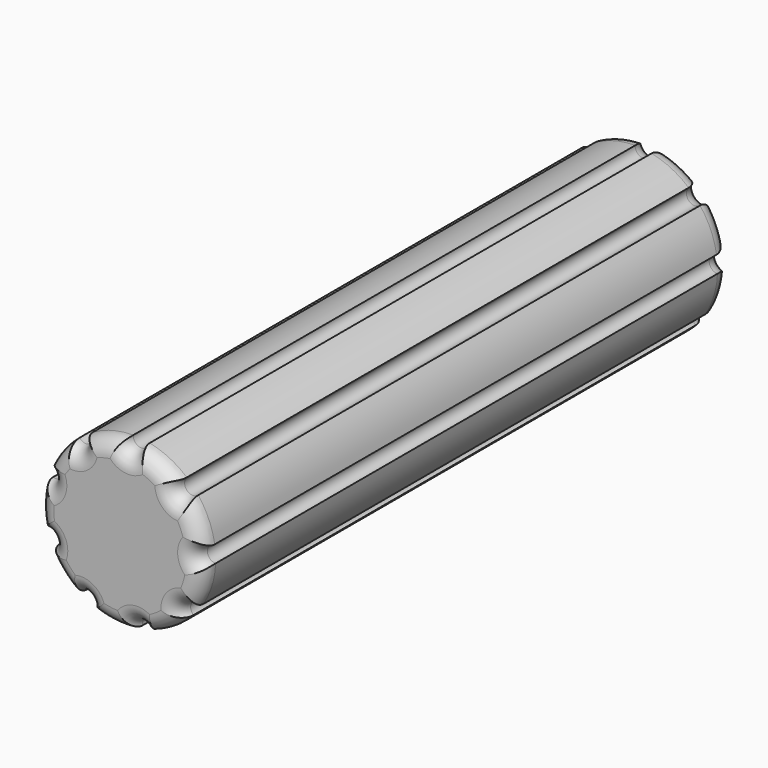
from build123d import *

# Parameters (mm, degrees)
F1_DEPTH     = 20
F2_T2_ANGLE  = 359.64
F2_T4_ANGLE  = 86.3342386314
F2_T6_ANGLE  = 359.64
F2_T8_ANGLE  = 86.3342386315
F2_T10_ANGLE = 359.64
F2_T12_ANGLE = 86.3342386314
F2_T14_ANGLE = 359.64
F2_T16_ANGLE = 81.8335537753
F2_T18_ANGLE = 359.64
F2_T20_ANGLE = 86.3342386314
F2_T22_ANGLE = 359.64
F2_T24_ANGLE = 86.3342386315
F2_T26_ANGLE = 359.64
F2_T28_ANGLE = 86.3342386315
F2_T30_ANGLE = 359.64
F2_T32_ANGLE = 86.3342386315
F2_T34_ANGLE = 359.64
F2_T36_ANGLE = 86.3342386315
F3_T2_ANGLE  = 359.64
F3_T4_ANGLE  = 86.3342386314
F3_T6_ANGLE  = 359.64
F3_T8_ANGLE  = 86.3342386315
F3_T10_ANGLE = 359.64
F3_T12_ANGLE = 86.3342386314
F3_T14_ANGLE = 359.64
F3_T16_ANGLE = 81.8335537753
F3_T18_ANGLE = 359.64
F3_T20_ANGLE = 86.3342386314
F3_T22_ANGLE = 359.64
F3_T24_ANGLE = 86.3342386315
F3_T26_ANGLE = 359.64
F3_T28_ANGLE = 86.3342386315
F3_T30_ANGLE = 359.64
F3_T32_ANGLE = 86.3342386315
F3_T34_ANGLE = 359.64
F3_T36_ANGLE = 86.3342386315


# Not quite as in the source:
# - a fillet or chamfer that OpenCascade refuses, or shapes differently, is made with other operations: its cross-section is extruded or revolved along the edge and cut away or added


with BuildPart() as f1:
    # F0 (on Front) → F1 (new body)
    with BuildSketch(Plane.XZ):
        with BuildLine():
            ThreePointArc((2.4975872126, -0.1098094511), (2.2464598382, 0.1261673312), (2.4695850963, 0.3887794391))
            ThreePointArc((2.4695850963, 0.3887794391), (2.2932672125, 0.9954524056), (1.9704957498, 1.538553379))
            ThreePointArc((1.9704957498, 1.538553379), (1.6262823354, 1.5548973489), (1.6253951918, 1.8994974258))
            ThreePointArc((1.6253951918, 1.8994974258), (1.0973194471, 2.2463058632), (0.4991662341, 2.4496597867))
            ThreePointArc((0.4991662341, 2.4496597867), (0.226809741, 2.2385391087), (0.0023353043, 2.4999989093))
            ThreePointArc((0.0023353043, 2.4999989093), (-0.6244507051, 2.4207563522), (-1.2113577854, 2.186918452))
            ThreePointArc((-1.2113577854, 2.186918452), (-1.1833130037, 2.1235912129), (-1.1737193058, 2.0549995957))
            ThreePointArc((-1.1737193058, 2.0549995957), (-1.3431931666, 1.8183235705), (-1.6218436331, 1.9025307434))
            ThreePointArc((-1.6218436331, 1.9025307434), (-1.9890673216, 1.5144672958), (-2.2654474487, 1.0572359515))
            ThreePointArc((-2.2654474487, 1.0572359515), (-2.1522675647, 0.9652125224), (-2.1097115694, 0.825688385))
            ThreePointArc((-2.1097115694, 0.825688385), (-2.2099897461, 0.6254800545), (-2.4303785744, 0.5858839347))
            ThreePointArc((-2.4303785744, 0.5858839347), (-2.4996457836, -0.0420827349), (-2.4092795801, -0.6673618996))
            ThreePointArc((-2.4092795801, -0.6673618996), (-2.1842499806, -0.7019514544), (-2.0805804647, -0.9046516997))
            ThreePointArc((-2.0805804647, -0.9046516997), (-2.1208172291, -1.0406641439), (-2.2285755446, -1.1328949828))
            ThreePointArc((-2.2285755446, -1.1328949828), (-1.8734150157, -1.6553900384), (-1.3986136823, -2.0721678908))
            ThreePointArc((-1.3986136823, -2.0721678908), (-1.1175350279, -1.9606743931), (-0.9346630079, -2.2014934835))
            ThreePointArc((-0.9346630079, -2.2014934835), (-0.9407887307, -2.2564965465), (-0.9588657034, -2.3088041413))
            ThreePointArc((-0.9588657034, -2.3088041413), (-0.3494661243, -2.4754541862), (0.2822512049, -2.4840157522))
            ThreePointArc((0.2822512049, -2.4840157522), (0.476037745, -2.1990652708), (0.7703211425, -2.3783619021))
            ThreePointArc((0.7703211425, -2.3783619021), (1.3419427643, -2.1093102231), (1.8278646823, -1.7055529025))
            ThreePointArc((1.8278646823, -1.7055529025), (1.7901605895, -1.3630205662), (2.1303792877, -1.3082370162))
            ThreePointArc((2.1303792877, -1.3082370162), (2.3903086912, -0.7324099678), (2.4975872126, -0.1098094511))
        make_face()
    extrude(amount=F1_DEPTH)

    # F2: fillet of radius 0.5 on 18 edges, made by hand

    # F2_s1 → F2_t2 (revolve, cut)
    with BuildSketch(Plane(origin=(-0.0004157691, 0, 0.0078429561), x_dir=(0, 1, 0), z_dir=(-0.0529374482, 0, 0.9985978302))):
        with BuildLine():
            ThreePointArc((-19.5, -2.749987663), (-19.8535533906, -2.8964342724), (-20, -3.249987663))
            Line((-20, -3.249987663), (-20, -2.749987663))
            Line((-20, -2.749987663), (-19.5, -2.749987663))
        make_face()
    revolve(axis=Axis((2.4960664869, -20, 0.1401859236), (0, 1, 0)), revolution_arc=F2_T2_ANGLE, mode=Mode.SUBTRACT)

    # F2_s3 → F2_t4 (revolve, cut)
    with BuildSketch(Plane(origin=(0, 0, 0), x_dir=(0, 1, 0), z_dir=(-0.3371381207, 0, -0.9414551968))):
        with BuildLine():
            ThreePointArc((-20, 2), (-19.8535533906, 2.3535533906), (-19.5, 2.5))
            Line((-19.5, 2.5), (-20, 2.5))
            Line((-20, 2.5), (-20, 2))
        make_face()
    revolve(axis=Axis((0, -20, 0), (0, -1, 0)), revolution_arc=F2_T4_ANGLE, mode=Mode.SUBTRACT)

    # F2_s5 → F2_t6 (revolve, cut)
    with BuildSketch(Plane(origin=(-0.0054097458, 0, 0.0056938102), x_dir=(0, 1, 0), z_dir=(-0.6887913634, 0, 0.7249596249))):
        with BuildLine():
            ThreePointArc((-20, -3.249987663), (-19.8535533906, -2.8964342724), (-19.5, -2.749987663))
            Line((-19.5, -2.749987663), (-20, -2.749987663))
            Line((-20, -2.749987663), (-20, -3.249987663))
        make_face()
    revolve(axis=Axis((1.8069803727, -20, 1.727663721), (0, 1, 0)), revolution_arc=F2_T6_ANGLE, mode=Mode.SUBTRACT)

    # F2_s7 → F2_t8 (revolve, cut)
    with BuildSketch(Plane(origin=(0, 0, 0), x_dir=(0, 1, 0), z_dir=(0.355064402, 0, -0.9348418425))):
        with BuildLine():
            ThreePointArc((-20, 2), (-19.8535533906, 2.3535533906), (-19.5, 2.5))
            Line((-19.5, 2.5), (-20, 2.5))
            Line((-20, 2.5), (-20, 2))
        make_face()
    revolve(axis=Axis((0, -20, 0), (0, -1, 0)), revolution_arc=F2_T8_ANGLE, mode=Mode.SUBTRACT)

    # F2_s9 → F2_t10 (revolve, cut)
    with BuildSketch(Plane(origin=(-0.0078114369, 0, 0.0008162584), x_dir=(0, 1, 0), z_dir=(-0.9945846753, 0, 0.103929417))):
        with BuildLine():
            ThreePointArc((-20, -3.249987663), (-19.8535533906, -2.8964342724), (-19.5, -2.749987663))
            Line((-19.5, -2.749987663), (-20, -2.749987663))
            Line((-20, -2.749987663), (-20, -3.249987663))
        make_face()
    revolve(axis=Axis((0.2520108233, -20, 2.4872656764), (0, 1, 0)), revolution_arc=F2_T10_ANGLE, mode=Mode.SUBTRACT)

    # F2_s11 → F2_t12 (revolve, cut)
    with BuildSketch(Plane(origin=(0, 0, 0), x_dir=(0, 1, 0), z_dir=(0.8771242995, 0, -0.480263431))):
        with BuildLine():
            ThreePointArc((-20, 2), (-19.8535533906, 2.3535533906), (-19.5, 2.5))
            Line((-19.5, 2.5), (-20, 2.5))
            Line((-20, 2.5), (-20, 2))
        make_face()
    revolve(axis=Axis((0, -20, 0), (0, -1, 0)), revolution_arc=F2_T12_ANGLE, mode=Mode.SUBTRACT)

    # F2_s13 → F2_t14 (revolve, cut)
    with BuildSketch(Plane(origin=(0.0064418777, 0, 0.0044929986), x_dir=(0, 1, 0), z_dir=(0.8202066864, 0, 0.5720672964))):
        with BuildLine():
            ThreePointArc((-20, 3.249987663), (-19.8535533906, 2.8964342724), (-19.5, 2.749987663))
            Line((-19.5, 2.749987663), (-20, 2.749987663))
            Line((-20, 2.749987663), (-20, 3.249987663))
        make_face()
    revolve(axis=Axis((-1.4237193058, -20, 2.0549995957), (0, -1, 0)), revolution_arc=F2_T14_ANGLE, mode=Mode.SUBTRACT)

    # F2_s15 → F2_t16 (revolve, cut)
    with BuildSketch(Plane(origin=(0, 0, 0), x_dir=(0, 1, 0), z_dir=(0.978875476, 0, 0.2044573367))):
        with BuildLine():
            ThreePointArc((-20, 2), (-19.8535533906, 2.3535533906), (-19.5, 2.5))
            Line((-19.5, 2.5), (-20, 2.5))
            Line((-20, 2.5), (-20, 2))
        make_face()
    revolve(axis=Axis((0, -20, 0), (0, -1, 0)), revolution_arc=F2_T16_ANGLE, mode=Mode.SUBTRACT)

    # F2_s17 → F2_t18 (revolve, cut)
    with BuildSketch(Plane(origin=(0.0025706702, 0, 0.0074213529), x_dir=(0, 1, 0), z_dir=(0.327308428, 0, 0.9449175588))):
        with BuildLine():
            ThreePointArc((-20, 3.249987663), (-19.8535533906, 2.8964342724), (-19.5, 2.749987663))
            Line((-19.5, 2.749987663), (-20, 2.749987663))
            Line((-20, 2.749987663), (-20, 3.249987663))
        make_face()
    revolve(axis=Axis((-2.3597115694, -20, 0.825688385), (0, -1, 0)), revolution_arc=F2_T18_ANGLE, mode=Mode.SUBTRACT)

    # F2_s19 → F2_t20 (revolve, cut)
    with BuildSketch(Plane(origin=(0, 0, 0), x_dir=(0, 1, 0), z_dir=(0.6717543155, 0, 0.7407740139))):
        with BuildLine():
            ThreePointArc((-20, 2), (-19.8535533906, 2.3535533906), (-19.5, 2.5))
            Line((-19.5, 2.5), (-20, 2.5))
            Line((-20, 2.5), (-20, 2))
        make_face()
    revolve(axis=Axis((0, -20, 0), (0, -1, 0)), revolution_arc=F2_T20_ANGLE, mode=Mode.SUBTRACT)

    # F2_s21 → F2_t22 (revolve, cut)
    with BuildSketch(Plane(origin=(-0.0028650303, 0, 0.0073127578), x_dir=(0, 1, 0), z_dir=(-0.3647875831, 0, 0.9310907685))):
        with BuildLine():
            ThreePointArc((-20, 3.249987663), (-19.8535533906, 2.8964342724), (-19.5, 2.749987663))
            Line((-19.5, 2.749987663), (-20, 2.749987663))
            Line((-20, 2.749987663), (-20, 3.249987663))
        make_face()
    revolve(axis=Axis((-2.3305804647, -20, -0.9046516997), (0, -1, 0)), revolution_arc=F2_T22_ANGLE, mode=Mode.SUBTRACT)

    # F2_s23 → F2_t24 (revolve, cut)
    with BuildSketch(Plane(origin=(0, 0, 0), x_dir=(0, 1, 0), z_dir=(0.0297117513, 0, 0.9995585085))):
        with BuildLine():
            ThreePointArc((-20, 2), (-19.8535533906, 2.3535533906), (-19.5, 2.5))
            Line((-19.5, 2.5), (-20, 2.5))
            Line((-20, 2.5), (-20, 2))
        make_face()
    revolve(axis=Axis((0, -20, 0), (0, -1, 0)), revolution_arc=F2_T24_ANGLE, mode=Mode.SUBTRACT)

    # F2_s25 → F2_t26 (revolve, cut)
    with BuildSketch(Plane(origin=(-0.0069278424, 0, 0.0036999763), x_dir=(0, 1, 0), z_dir=(-0.8820817368, 0, 0.471096391))):
        with BuildLine():
            ThreePointArc((-20, 3.249987663), (-19.8535533906, 2.8964342724), (-19.5, 2.749987663))
            Line((-19.5, 2.749987663), (-20, 2.749987663))
            Line((-20, 2.749987663), (-20, 3.249987663))
        make_face()
    revolve(axis=Axis((-1.1846630079, -20, -2.2014934835), (0, -1, 0)), revolution_arc=F2_T26_ANGLE, mode=Mode.SUBTRACT)

    # F2_s27 → F2_t28 (revolve, cut)
    with BuildSketch(Plane(origin=(0, 0, 0), x_dir=(0, 1, 0), z_dir=(-0.6265683296, 0, 0.7793664917))):
        with BuildLine():
            ThreePointArc((-20, 2), (-19.8535533906, 2.3535533906), (-19.5, 2.5))
            Line((-19.5, 2.5), (-20, 2.5))
            Line((-20, 2.5), (-20, 2))
        make_face()
    revolve(axis=Axis((0, -20, 0), (0, -1, 0)), revolution_arc=F2_T28_ANGLE, mode=Mode.SUBTRACT)

    # F2_s29 → F2_t30 (revolve, cut)
    with BuildSketch(Plane(origin=(0.0076813557, 0, 0.0016375589), x_dir=(0, 1, 0), z_dir=(0.9780221925, 0, 0.2085008178))):
        with BuildLine():
            ThreePointArc((-20, -3.249987663), (-19.8535533906, -2.8964342724), (-19.5, -2.749987663))
            Line((-19.5, -2.749987663), (-20, -2.749987663))
            Line((-20, -2.749987663), (-20, -3.249987663))
        make_face()
    revolve(axis=Axis((0.5289308278, -20, -2.4434058565), (0, 1, 0)), revolution_arc=F2_T30_ANGLE, mode=Mode.SUBTRACT)

    # F2_s31 → F2_t32 (revolve, cut)
    with BuildSketch(Plane(origin=(0, 0, 0), x_dir=(0, 1, 0), z_dir=(-0.9826043426, 0, 0.1857113509))):
        with BuildLine():
            ThreePointArc((-20, 2), (-19.8535533906, 2.3535533906), (-19.5, 2.5))
            Line((-19.5, 2.5), (-20, 2.5))
            Line((-20, 2.5), (-20, 2))
        make_face()
    revolve(axis=Axis((0, -20, 0), (0, -1, 0)), revolution_arc=F2_T32_ANGLE, mode=Mode.SUBTRACT)

    # F2_s33 → F2_t34 (revolve, cut)
    with BuildSketch(Plane(origin=(0.0047774393, 0, 0.006233851), x_dir=(0, 1, 0), z_dir=(0.6082834605, 0, 0.7937198698))):
        with BuildLine():
            ThreePointArc((-20, -3.249987663), (-19.8535533906, -2.8964342724), (-19.5, -2.749987663))
            Line((-19.5, -2.749987663), (-20, -2.749987663))
            Line((-20, -2.749987663), (-20, -3.249987663))
        make_face()
    revolve(axis=Axis((1.9890673216, -20, -1.5144672958), (0, 1, 0)), revolution_arc=F2_T34_ANGLE, mode=Mode.SUBTRACT)

    # F2_s35 → F2_t36 (revolve, cut)
    with BuildSketch(Plane(origin=(0, 0, 0), x_dir=(0, 1, 0), z_dir=(-0.8677880783, 0, -0.4969344535))):
        with BuildLine():
            ThreePointArc((-20, 2), (-19.8535533906, 2.3535533906), (-19.5, 2.5))
            Line((-19.5, 2.5), (-20, 2.5))
            Line((-20, 2.5), (-20, 2))
        make_face()
    revolve(axis=Axis((0, -20, 0), (0, -1, 0)), revolution_arc=F2_T36_ANGLE, mode=Mode.SUBTRACT)

    # F3: fillet of radius 0.5 on 18 edges, made by hand

    # F3_s1 → F3_t2 (revolve, cut)
    with BuildSketch(Plane(origin=(-0.0004157691, 0, 0.0078429561), x_dir=(0, 1, 0), z_dir=(-0.0529374482, 0, 0.9985978302))):
        with BuildLine():
            ThreePointArc((-0.5, -2.749987663), (-0.1464466094, -2.8964342724), (0, -3.249987663))
            Line((0, -3.249987663), (0, -2.749987663))
            Line((0, -2.749987663), (-0.5, -2.749987663))
        make_face()
    revolve(axis=Axis((2.4960664869, 0, 0.1401859236), (0, 1, 0)), revolution_arc=F3_T2_ANGLE, mode=Mode.SUBTRACT)

    # F3_s3 → F3_t4 (revolve, cut)
    with BuildSketch(Plane(origin=(0, 0, 0), x_dir=(0, 1, 0), z_dir=(-0.3371381207, 0, -0.9414551968))):
        with BuildLine():
            ThreePointArc((-0.5, 2.5), (-0.1464466094, 2.3535533906), (0, 2))
            Line((0, 2), (0, 2.5))
            Line((0, 2.5), (-0.5, 2.5))
        make_face()
    revolve(axis=Axis((0, 0, 0), (0, -1, 0)), revolution_arc=F3_T4_ANGLE, mode=Mode.SUBTRACT)

    # F3_s5 → F3_t6 (revolve, cut)
    with BuildSketch(Plane(origin=(-0.0054097458, 0, 0.0056938102), x_dir=(0, 1, 0), z_dir=(-0.6887913634, 0, 0.7249596249))):
        with BuildLine():
            ThreePointArc((-0.5, -2.749987663), (-0.1464466094, -2.8964342724), (0, -3.249987663))
            Line((0, -3.249987663), (0, -2.749987663))
            Line((0, -2.749987663), (-0.5, -2.749987663))
        make_face()
    revolve(axis=Axis((1.8069803727, 0, 1.727663721), (0, 1, 0)), revolution_arc=F3_T6_ANGLE, mode=Mode.SUBTRACT)

    # F3_s7 → F3_t8 (revolve, cut)
    with BuildSketch(Plane(origin=(0, 0, 0), x_dir=(0, 1, 0), z_dir=(0.355064402, 0, -0.9348418425))):
        with BuildLine():
            ThreePointArc((-0.5, 2.5), (-0.1464466094, 2.3535533906), (0, 2))
            Line((0, 2), (0, 2.5))
            Line((0, 2.5), (-0.5, 2.5))
        make_face()
    revolve(axis=Axis((0, 0, 0), (0, -1, 0)), revolution_arc=F3_T8_ANGLE, mode=Mode.SUBTRACT)

    # F3_s9 → F3_t10 (revolve, cut)
    with BuildSketch(Plane(origin=(-0.0078114369, 0, 0.0008162584), x_dir=(0, 1, 0), z_dir=(-0.9945846753, 0, 0.103929417))):
        with BuildLine():
            ThreePointArc((-0.5, -2.749987663), (-0.1464466094, -2.8964342724), (0, -3.249987663))
            Line((0, -3.249987663), (0, -2.749987663))
            Line((0, -2.749987663), (-0.5, -2.749987663))
        make_face()
    revolve(axis=Axis((0.2520108233, 0, 2.4872656764), (0, 1, 0)), revolution_arc=F3_T10_ANGLE, mode=Mode.SUBTRACT)

    # F3_s11 → F3_t12 (revolve, cut)
    with BuildSketch(Plane(origin=(0, 0, 0), x_dir=(0, 1, 0), z_dir=(0.8771242995, 0, -0.480263431))):
        with BuildLine():
            ThreePointArc((-0.5, 2.5), (-0.1464466094, 2.3535533906), (0, 2))
            Line((0, 2), (0, 2.5))
            Line((0, 2.5), (-0.5, 2.5))
        make_face()
    revolve(axis=Axis((0, 0, 0), (0, -1, 0)), revolution_arc=F3_T12_ANGLE, mode=Mode.SUBTRACT)

    # F3_s13 → F3_t14 (revolve, cut)
    with BuildSketch(Plane(origin=(-0.0064699807, 0, -0.0044524347), x_dir=(0, 1, 0), z_dir=(-0.8237848774, 0, -0.5669025276))):
        with BuildLine():
            ThreePointArc((-0.5, -2.749987663), (-0.1464466094, -2.8964342724), (0, -3.249987663))
            Line((0, -3.249987663), (0, -2.749987663))
            Line((0, -2.749987663), (-0.5, -2.749987663))
        make_face()
    revolve(axis=Axis((-1.4237193058, 0, 2.0549995957), (0, 1, 0)), revolution_arc=F3_T14_ANGLE, mode=Mode.SUBTRACT)

    # F3_s15 → F3_t16 (revolve, cut)
    with BuildSketch(Plane(origin=(0, 0, 0), x_dir=(0, 1, 0), z_dir=(0.978875476, 0, 0.2044573367))):
        with BuildLine():
            ThreePointArc((-0.5, 2.5), (-0.1464466094, 2.3535533906), (0, 2))
            Line((0, 2), (0, 2.5))
            Line((0, 2.5), (-0.5, 2.5))
        make_face()
    revolve(axis=Axis((0, 0, 0), (0, -1, 0)), revolution_arc=F3_T16_ANGLE, mode=Mode.SUBTRACT)

    # F3_s17 → F3_t18 (revolve, cut)
    with BuildSketch(Plane(origin=(-0.0026172488, 0, -0.0074050546), x_dir=(0, 1, 0), z_dir=(-0.3332390203, 0, -0.942842381))):
        with BuildLine():
            ThreePointArc((-0.5, -2.749987663), (-0.1464466094, -2.8964342724), (0, -3.249987663))
            Line((0, -3.249987663), (0, -2.749987663))
            Line((0, -2.749987663), (-0.5, -2.749987663))
        make_face()
    revolve(axis=Axis((-2.3597115694, 0, 0.825688385), (0, 1, 0)), revolution_arc=F3_T18_ANGLE, mode=Mode.SUBTRACT)

    # F3_s19 → F3_t20 (revolve, cut)
    with BuildSketch(Plane(origin=(0, 0, 0), x_dir=(0, 1, 0), z_dir=(0.6717543155, 0, 0.7407740139))):
        with BuildLine():
            ThreePointArc((-0.5, 2.5), (-0.1464466094, 2.3535533906), (0, 2))
            Line((0, 2), (0, 2.5))
            Line((0, 2.5), (-0.5, 2.5))
        make_face()
    revolve(axis=Axis((0, 0, 0), (0, -1, 0)), revolution_arc=F3_T20_ANGLE, mode=Mode.SUBTRACT)

    # F3_s21 → F3_t22 (revolve, cut)
    with BuildSketch(Plane(origin=(0.0028190266, 0, -0.0073306148), x_dir=(0, 1, 0), z_dir=(0.3589302052, 0, -0.9333644025))):
        with BuildLine():
            ThreePointArc((-0.5, -2.749987663), (-0.1464466094, -2.8964342724), (0, -3.249987663))
            Line((0, -3.249987663), (0, -2.749987663))
            Line((0, -2.749987663), (-0.5, -2.749987663))
        make_face()
    revolve(axis=Axis((-2.3305804647, 0, -0.9046516997), (0, 1, 0)), revolution_arc=F3_T22_ANGLE, mode=Mode.SUBTRACT)

    # F3_s23 → F3_t24 (revolve, cut)
    with BuildSketch(Plane(origin=(0, 0, 0), x_dir=(0, 1, 0), z_dir=(0.0297117513, 0, 0.9995585085))):
        with BuildLine():
            ThreePointArc((-0.5, 2.5), (-0.1464466094, 2.3535533906), (0, 2))
            Line((0, 2), (0, 2.5))
            Line((0, 2.5), (-0.5, 2.5))
        make_face()
    revolve(axis=Axis((0, 0, 0), (0, -1, 0)), revolution_arc=F3_T24_ANGLE, mode=Mode.SUBTRACT)

    # F3_s25 → F3_t26 (revolve, cut)
    with BuildSketch(Plane(origin=(0.0069044581, 0, -0.0037434319), x_dir=(0, 1, 0), z_dir=(0.8791043588, 0, -0.4766293385))):
        with BuildLine():
            ThreePointArc((-0.5, -2.749987663), (-0.1464466094, -2.8964342724), (0, -3.249987663))
            Line((0, -3.249987663), (0, -2.749987663))
            Line((0, -2.749987663), (-0.5, -2.749987663))
        make_face()
    revolve(axis=Axis((-1.1846630079, 0, -2.2014934835), (0, 1, 0)), revolution_arc=F3_T26_ANGLE, mode=Mode.SUBTRACT)

    # F3_s27 → F3_t28 (revolve, cut)
    with BuildSketch(Plane(origin=(0, 0, 0), x_dir=(0, 1, 0), z_dir=(-0.6265683296, 0, 0.7793664917))):
        with BuildLine():
            ThreePointArc((-0.5, 2.5), (-0.1464466094, 2.3535533906), (0, 2))
            Line((0, 2), (0, 2.5))
            Line((0, 2.5), (-0.5, 2.5))
        make_face()
    revolve(axis=Axis((0, 0, 0), (0, -1, 0)), revolution_arc=F3_T28_ANGLE, mode=Mode.SUBTRACT)

    # F3_s29 → F3_t30 (revolve, cut)
    with BuildSketch(Plane(origin=(0.0076813557, 0, 0.0016375589), x_dir=(0, 1, 0), z_dir=(0.9780221925, 0, 0.2085008178))):
        with BuildLine():
            ThreePointArc((-0.5, -2.749987663), (-0.1464466094, -2.8964342724), (0, -3.249987663))
            Line((0, -3.249987663), (0, -2.749987663))
            Line((0, -2.749987663), (-0.5, -2.749987663))
        make_face()
    revolve(axis=Axis((0.5289308278, 0, -2.4434058565), (0, 1, 0)), revolution_arc=F3_T30_ANGLE, mode=Mode.SUBTRACT)

    # F3_s31 → F3_t32 (revolve, cut)
    with BuildSketch(Plane(origin=(0, 0, 0), x_dir=(0, 1, 0), z_dir=(-0.9826043426, 0, 0.1857113509))):
        with BuildLine():
            ThreePointArc((-0.5, 2.5), (-0.1464466094, 2.3535533906), (0, 2))
            Line((0, 2), (0, 2.5))
            Line((0, 2.5), (-0.5, 2.5))
        make_face()
    revolve(axis=Axis((0, 0, 0), (0, -1, 0)), revolution_arc=F3_T32_ANGLE, mode=Mode.SUBTRACT)

    # F3_s33 → F3_t34 (revolve, cut)
    with BuildSketch(Plane(origin=(0.0047774393, 0, 0.006233851), x_dir=(0, 1, 0), z_dir=(0.6082834605, 0, 0.7937198698))):
        with BuildLine():
            ThreePointArc((-0.5, -2.749987663), (-0.1464466094, -2.8964342724), (0, -3.249987663))
            Line((0, -3.249987663), (0, -2.749987663))
            Line((0, -2.749987663), (-0.5, -2.749987663))
        make_face()
    revolve(axis=Axis((1.9890673216, 0, -1.5144672958), (0, 1, 0)), revolution_arc=F3_T34_ANGLE, mode=Mode.SUBTRACT)

    # F3_s35 → F3_t36 (revolve, cut)
    with BuildSketch(Plane(origin=(0, 0, 0), x_dir=(0, 1, 0), z_dir=(-0.8677880783, 0, -0.4969344535))):
        with BuildLine():
            ThreePointArc((-0.5, 2.5), (-0.1464466094, 2.3535533906), (0, 2))
            Line((0, 2), (0, 2.5))
            Line((0, 2.5), (-0.5, 2.5))
        make_face()
    revolve(axis=Axis((0, 0, 0), (0, -1, 0)), revolution_arc=F3_T36_ANGLE, mode=Mode.SUBTRACT)


solid = f1.part
